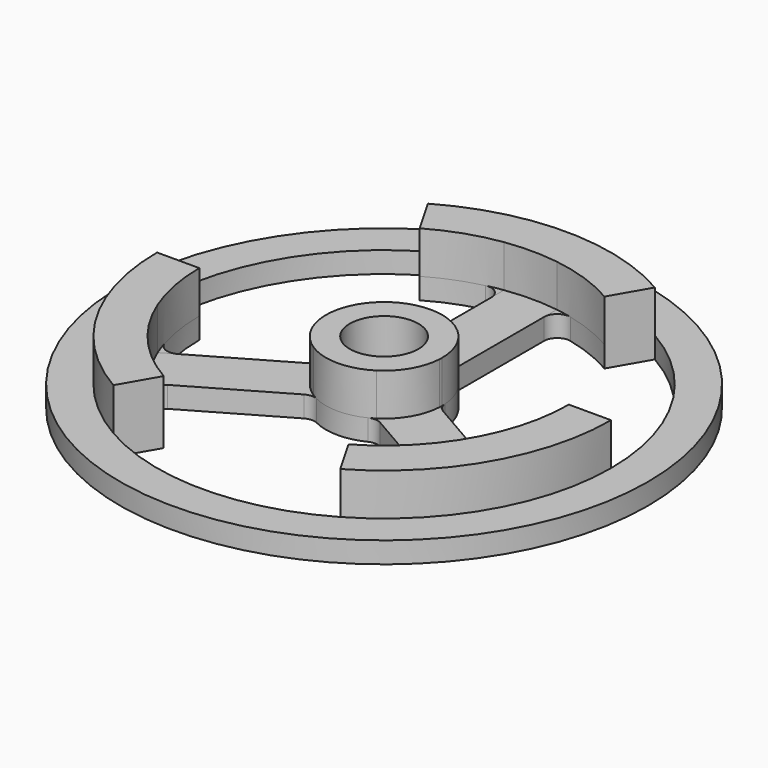
from build123d import *
from build123d import SkipClean  # not in build123d's __all__

# Parameters (mm, degrees)
F0_R          = 31.75
F1_DEPTH      = 2.54
F2_R          = 27.305
F2_R_2        = 22.225
F2_R_3        = 6.985
F3_DEPTH      = 5.08
F4_R          = 4.1275
F5_DEPTH      = 25.4
F5_DEPTH_BACK = 96
F7_DEPTH      = 25.4
F7_DEPTH_BACK = 5.081
F8_T1_DEPTH   = 2.54
F10_DEPTH     = 25.4


# Not quite as in the source:
# - a fillet or chamfer that OpenCascade refuses, or shapes differently, is made with other operations: its cross-section is extruded or revolved along the edge and cut away or added
# - an extrude ends at something that could not be found from the text; its depth is read off the source's solid


with BuildPart() as f1:
    # F0 (on Top) → F1 (new body)
    with BuildSketch(Plane.XY):
        Circle(F0_R)
    extrude(amount=F1_DEPTH)

    # F2 (on face) → F3 (join)
    with BuildSketch(Plane.XY.offset(2.54)):
        Circle(F2_R)
        Circle(F2_R_2, mode=Mode.SUBTRACT)
        Circle(F2_R_3)
    extrude(amount=F3_DEPTH)

    # F4 (on face) → F5 (cut, two sides)
    with BuildSketch(Plane.XY.offset(7.62)) as f5_sk:
        Circle(F4_R)
    extrude(amount=-F5_DEPTH, mode=Mode.SUBTRACT)
    extrude(f5_sk.sketch, amount=F5_DEPTH_BACK, mode=Mode.SUBTRACT)

    # F6 (on face) → F7 (cut, two sides)
    with BuildSketch(Plane.XY.offset(2.54)) as f7_sk:
        with BuildLine():
            Line((3.175, 21.9970452561), (3.175, 6.2217039467))
            ThreePointArc((3.175, 6.2217039467), (5.956828015, 3.6477972806), (6.985, 0))
            ThreePointArc((6.985, 0), (6.9826630272, -0.1806711053), (6.9756536726, -0.3612213163))
            Line((6.9756536726, -0.3612213163), (20.6375, -8.248891971))
            ThreePointArc((20.6375, -8.248891971), (21.8245167472, -4.2001302063), (22.225, 0))
            ThreePointArc((22.225, 0), (16.8005208253, 14.5496778315), (3.175, 21.9970452561))
        make_face()
        with BuildLine():
            Line((17.4625, -13.7481532851), (3.8006536726, -5.8604826304))
            ThreePointArc((3.8006536726, -5.8604826304), (0, -6.985), (-3.8006536726, -5.8604826304))
            Line((-3.8006536726, -5.8604826304), (-17.4625, -13.7481532851))
            ThreePointArc((-17.4625, -13.7481532851), (0, -22.225), (17.4625, -13.7481532851))
        make_face()
        with BuildLine():
            ThreePointArc((-6.9756536726, -0.3612213163), (-6.0491874454, 3.4925), (-3.175, 6.2217039467))
            Line((-3.175, 6.2217039467), (-3.175, 21.9970452561))
            ThreePointArc((-3.175, 21.9970452561), (-19.2474145991, 11.1125), (-20.6375, -8.248891971))
            Line((-20.6375, -8.248891971), (-6.9756536726, -0.3612213163))
        make_face()
    with SkipClean():  # cleaning this boolean's faces spoils the solid; the shape is the same uncleaned
        extrude(amount=-F7_DEPTH, mode=Mode.SUBTRACT)
        extrude(f7_sk.sketch, amount=F7_DEPTH_BACK, mode=Mode.SUBTRACT)

    # F8: fillet of radius 1.5875 on 18 edges, made by hand

    # F8_s2 → F8_t1 (join)
    with BuildSketch(Plane.XY):
        with BuildLine():
            ThreePointArc((16.1634751393, -15.2542681378), (16.5796979287, -13.9347220137), (15.8026912008, -12.7898622281))
            Line((15.8026912008, -12.7898622281), (17.4625, -13.7481532851))
            ThreePointArc((17.4625, -13.7481532851), (16.829843924, -14.515749326), (16.1634751393, -15.2542681378))
        make_face()
        with BuildLine():
            ThreePointArc((18.9776912008, -7.290600914), (20.3576722229, -7.3910785865), (21.2923212932, -6.3708460152))
            ThreePointArc((21.2923212932, -6.3708460152), (20.9859296333, -7.3171977169), (20.6375, -8.248891971))
            Line((20.6375, -8.248891971), (18.9776912008, -7.290600914))
        make_face()
        with BuildLine():
            ThreePointArc((3.175, 20.0804631421), (3.7779742942, 21.3258006002), (5.1288461538, 21.625114153))
            ThreePointArc((5.1288461538, 21.625114153), (4.1560857093, 21.8329470429), (3.175, 21.9970452561))
            Line((3.175, 21.9970452561), (3.175, 20.0804631421))
        make_face()
        with BuildLine():
            ThreePointArc((-3.175, 20.0804631421), (-3.7779742942, 21.3258006002), (-5.1288461538, 21.625114153))
            ThreePointArc((-5.1288461538, 21.625114153), (-4.1560857093, 21.8329470429), (-3.175, 21.9970452561))
            Line((-3.175, 21.9970452561), (-3.175, 20.0804631421))
        make_face()
        with BuildLine():
            ThreePointArc((-18.9776912008, -7.290600914), (-20.3576722229, -7.3910785865), (-21.2923212932, -6.3708460152))
            ThreePointArc((-21.2923212932, -6.3708460152), (-20.9859296333, -7.3171977169), (-20.6375, -8.248891971))
            Line((-20.6375, -8.248891971), (-18.9776912008, -7.290600914))
        make_face()
        with BuildLine():
            ThreePointArc((-16.1634751393, -15.2542681378), (-16.5796979287, -13.9347220137), (-15.8026912008, -12.7898622281))
            Line((-15.8026912008, -12.7898622281), (-17.4625, -13.7481532851))
            ThreePointArc((-17.4625, -13.7481532851), (-16.829843924, -14.515749326), (-16.1634751393, -15.2542681378))
        make_face()
        with BuildLine():
            ThreePointArc((4.5854055152, -6.3135593179), (3.8435830552, -6.1017241554), (3.0894970865, -6.2646015638))
            ThreePointArc((3.0894970865, -6.2646015638), (3.4509958561, -6.0729607772), (3.8006536726, -5.8604826304))
            Line((3.8006536726, -5.8604826304), (4.5854055152, -6.3135593179))
        make_face()
        with BuildLine():
            ThreePointArc((-3.0894970865, -6.2646015638), (-3.8435830552, -6.1017241554), (-4.5854055152, -6.3135593179))
            Line((-4.5854055152, -6.3135593179), (-3.8006536726, -5.8604826304))
            ThreePointArc((-3.8006536726, -5.8604826304), (-3.4509958561, -6.0729607772), (-3.0894970865, -6.2646015638))
        make_face()
        with BuildLine():
            ThreePointArc((-7.7604055152, -0.8142980039), (-7.2060396531, -0.2777784896), (-6.970052642, 0.4567178201))
            ThreePointArc((-6.970052642, 0.4567178201), (-6.9848362373, 0.0478303088), (-6.9756536726, -0.3612213163))
            Line((-6.9756536726, -0.3612213163), (-7.7604055152, -0.8142980039))
        make_face()
        with BuildLine():
            ThreePointArc((-3.8805555556, 5.8078837437), (-3.3624565979, 6.379502645), (-3.175, 7.1278573218))
            Line((-3.175, 7.1278573218), (-3.175, 6.2217039467))
            ThreePointArc((-3.175, 6.2217039467), (-3.5338403812, 6.0251304683), (-3.8805555556, 5.8078837437))
        make_face()
        with BuildLine():
            ThreePointArc((3.175, 7.1278573218), (3.3624565979, 6.379502645), (3.8805555556, 5.8078837437))
            ThreePointArc((3.8805555556, 5.8078837437), (3.5338403812, 6.0251304683), (3.175, 6.2217039467))
            Line((3.175, 6.2217039467), (3.175, 7.1278573218))
        make_face()
        with BuildLine():
            ThreePointArc((6.970052642, 0.4567178201), (7.2060396531, -0.2777784896), (7.7604055152, -0.8142980039))
            Line((7.7604055152, -0.8142980039), (6.9756536726, -0.3612213163))
            ThreePointArc((6.9756536726, -0.3612213163), (6.9848362373, 0.0478303088), (6.970052642, 0.4567178201))
        make_face()
    with SkipClean():  # cleaning this boolean's faces spoils the solid; the shape is the same uncleaned
        extrude(amount=F8_T1_DEPTH)

    # F9 (on face) → F10 (cut)
    with BuildSketch(Plane.XY.offset(7.62)):
        with BuildLine():
            ThreePointArc((27.305, 0), (23.6468236503, 13.6525), (13.6525, 23.6468236503))
            Line((13.6525, 23.6468236503), (11.1125, 19.2474145991))
            ThreePointArc((11.1125, 19.2474145991), (19.2474145991, 11.1125), (22.225, 0))
            Line((22.225, 0), (27.305, 0))
        make_face()
        with BuildLine():
            Line((-11.1125, -19.2474145991), (-13.6525, -23.6468236503))
            ThreePointArc((-13.6525, -23.6468236503), (0, -27.305), (13.6525, -23.6468236503))
            Line((13.6525, -23.6468236503), (11.1125, -19.2474145991))
            ThreePointArc((11.1125, -19.2474145991), (0, -22.225), (-11.1125, -19.2474145991))
        make_face()
        with BuildLine():
            ThreePointArc((-22.225, 0), (-19.2474145991, 11.1125), (-11.1125, 19.2474145991))
            Line((-11.1125, 19.2474145991), (-13.6525, 23.6468236503))
            ThreePointArc((-13.6525, 23.6468236503), (-23.6468236503, 13.6525), (-27.305, 0))
            Line((-27.305, 0), (-22.225, 0))
        make_face()
    with SkipClean():  # cleaning this boolean's faces spoils the solid; the shape is the same uncleaned
        extrude(amount=-F10_DEPTH, mode=Mode.SUBTRACT)


solid = f1.part
